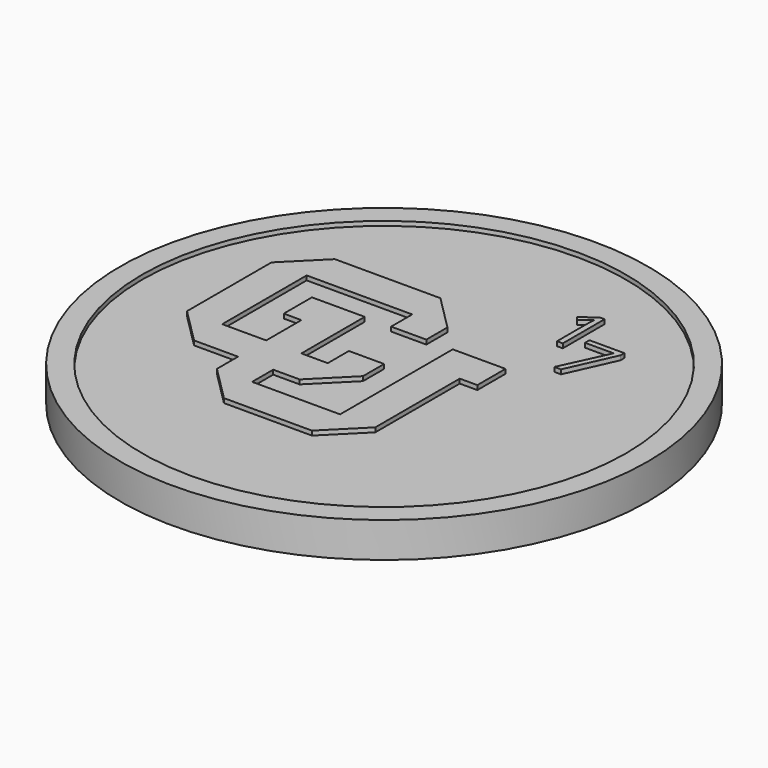
from build123d import *

# Parameters (mm, degrees)
F0_R         = 38.1
F1_DEPTH     = 3.81
F2_R         = 38.1
F2_R_2       = 34.925
F2_TEXT_SIZE = 10.5833333333
F3_DEPTH     = 0.635
F4_R         = 38.1
F4_R_2       = 34.925
F4_TEXT_SIZE = 14.1111111111
F5_DEPTH     = 0.635


# Not quite as in the source:
# - a feature names something its author has since deleted; it is built from what else it names
# - Text() gives the source's letters only with a copy of the font that has no kerning and outlines rounded to 1/6400 em; it was checked with that copy


with BuildPart() as f1:
    # F0 (on Top) → F1 (new body)
    with BuildSketch(Plane.XY):
        Circle(F0_R)
    extrude(amount=F1_DEPTH)

    # F2 (on face) → F3 (join)
    with BuildSketch(Plane.XY.offset(3.81)):
        Circle(F2_R)
        Circle(F2_R_2, mode=Mode.SUBTRACT)
        Polygon((0, -3.81), (0, 0), (-5.08, 0), (-5.08, -3.81), (-8.89, -3.81), (-8.89, 7.62), (-16.51, 7.62), (-16.51, 2.54), (-13.97, 2.54), (-13.97, -3.81), (-20.32, -3.81), (-20.32, 11.43), (-5.08, 11.43), (-5.08, 7.62), (0, 7.62), (0, 11.43), (-5.08, 16.51), (-20.32, 16.51), (-25.4, 11.43), (-25.4, -3.81), (-20.32, -8.89), (-13.97, -8.89), (-13.97, -12.7), (-8.89, -17.78), (3.81, -17.78), (8.89, -12.7), (8.89, 2.54), (11.43, 2.54), (11.43, 7.62), (3.81, 7.62), (3.81, -12.7), (-8.89, -12.7), (-8.89, -8.89), (-5.08, -8.89), align=None)
        with Locations((8.89, 16.51)):
            Text('1', F2_TEXT_SIZE, font='Open Sans', text_align=(TextAlign.LEFT, TextAlign.BOTTOM))
        with Locations((13.97, 11.43)):
            Text('7', F2_TEXT_SIZE, font='Open Sans', text_align=(TextAlign.LEFT, TextAlign.BOTTOM))
    extrude(amount=F3_DEPTH)

    # F4 (on face) → F5 (join)
    with BuildSketch(Plane(origin=(0, 0, 0), x_dir=(1, 0, 0), z_dir=(0, 0, -1))):
        Circle(F4_R)
        Circle(F4_R_2, mode=Mode.SUBTRACT)
        with Locations((-15.24, -12.7)):
            Text('Macias', F4_TEXT_SIZE, font='Open Sans', text_align=(TextAlign.LEFT, TextAlign.BOTTOM))
        with Locations((-25.4, 2.54)):
            Text('Jocelin', F4_TEXT_SIZE, font='Open Sans', text_align=(TextAlign.LEFT, TextAlign.BOTTOM))
    extrude(amount=F5_DEPTH)


solid = f1.part
